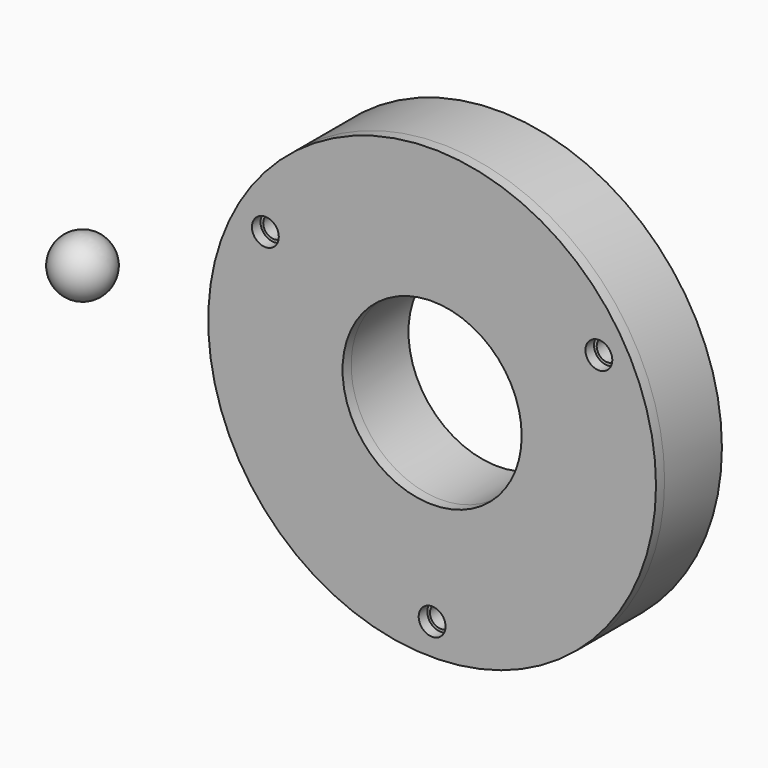
from build123d import *

# Parameters (mm, degrees)
F0_R            = 25
F0_R_2          = 10
F1_DEPTH        = 8
F3_DEPTH        = 6.5
F3_COPIES_COUNT = 3
F5_D            = 2.4
F5_COPIES_COUNT = 3
F6_R            = 25
F6_R_2          = 1.5
F6_R_3          = 10
F7_DEPTH        = 1.2


# Not quite as in the source:
# - a pattern or mirror of a feature is missing from the dataset's text; its kind, count and spacing are read off the source's solid


with BuildPart() as f1:
    # F0 (on Front) → F1 (new body)
    with BuildSketch(Plane.XZ):
        Circle(F0_R)
        Circle(F0_R_2, mode=Mode.SUBTRACT)
    extrude(amount=-F1_DEPTH)

    # F2 (on face) → F3 (cut)
    with BuildSketch(Plane.XZ):
        with BuildLine():
            ThreePointArc((-16.4402326626, 16.4402326626), (-16.4402326626, 11.8440385849), (-11.8440385849, 11.8440385849))
            ThreePointArc((-11.8440385849, 11.8440385849), (0, 16.75), (11.8440385849, 11.8440385849))
            ThreePointArc((11.8440385849, 11.8440385849), (16.4402326626, 11.8440385849), (16.4402326626, 16.4402326626))
            ThreePointArc((16.4402326626, 16.4402326626), (0, 23.25), (-16.4402326626, 16.4402326626))
        make_face()
    f3 = extrude(amount=-F3_DEPTH, mode=Mode.SUBTRACT)

    # F3_copies: F3 ×3 about axis
    f3_copies_axis = Axis((0, 0, 0), (0, 1, 0))
    for i in range(1, F3_COPIES_COUNT):
        add(f3.rotate(f3_copies_axis, i * 360 / F3_COPIES_COUNT), mode=Mode.SUBTRACT)

    # F5 (through all)
    with Locations(Plane.XZ):
        with Locations((0, -21.5)):
            f5 = Hole(F5_D / 2)

    # F5_copies: F5 ×3 about axis
    f5_copies_axis = Axis((0, 0, 0), (0, 1, 0))
    for i in range(1, F5_COPIES_COUNT):
        add(f5.rotate(f5_copies_axis, i * 360 / F5_COPIES_COUNT), mode=Mode.SUBTRACT)


with BuildPart() as f7:
    # F6 (on face) → F7 (new body)
    with BuildSketch(Plane.XZ):
        Circle(F6_R)
        with Locations((0, -21.5)):
            Circle(F6_R_2, mode=Mode.SUBTRACT)
        with Locations((-18.6195461814, 10.75)):
            Circle(F6_R_2, mode=Mode.SUBTRACT)
        Circle(F6_R_3, mode=Mode.SUBTRACT)
        with Locations((18.6195461814, 10.75)):
            Circle(F6_R_2, mode=Mode.SUBTRACT)
    extrude(amount=F7_DEPTH)


with BuildPart() as f9:
    # F8 (on Front) → F9 (revolve)
    with BuildSketch(Plane.XZ):
        with BuildLine():
            Line((-43.175, 0), (-36.825, 0))
            ThreePointArc((-36.825, 0), (-40, 3.175), (-43.175, 0))
        make_face()
    revolve(axis=Axis((-40, 0, 0), (1, 0, 0)))


solid = Compound([f1.part, f7.part, f9.part])
